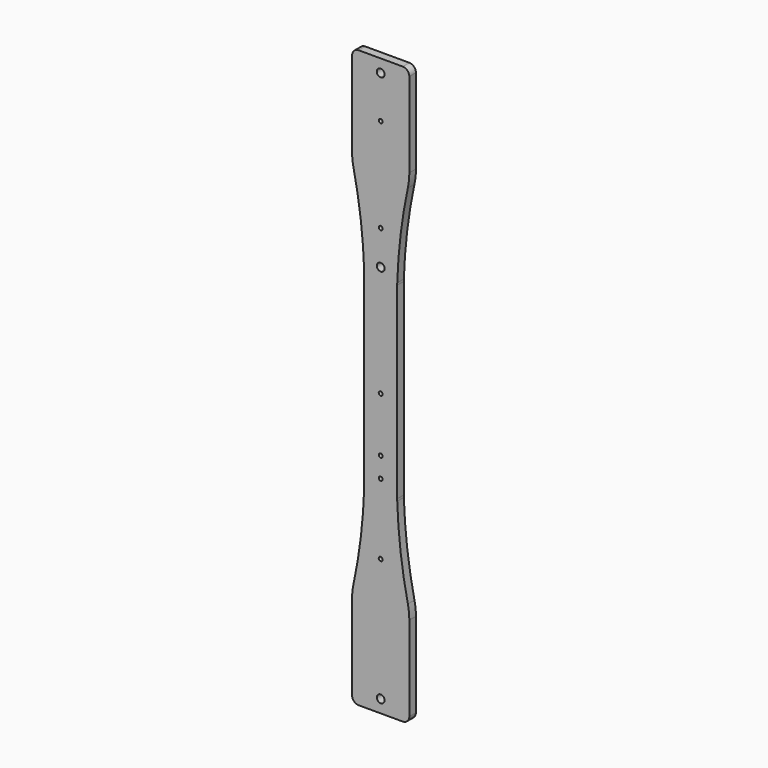
from build123d import *

# Parameters (mm, degrees)
F0_R        = 3
F0_R_2      = 1.5
F1_DEPTH    = 6.35
F2_R        = 5.08
F3_T1_DEPTH = 6.35
F3_T3_DEPTH = 34.0624500619


# Not quite as in the source:
# - a fillet or chamfer that OpenCascade refuses, or shapes differently, is made with other operations: its cross-section is extruded or revolved along the edge and cut away or added
# - a feature names something its author has since deleted; it is built from what else it names


with BuildPart() as f1:
    # F0 (on Front) → F1 (new body)
    with BuildSketch(Plane.XZ):
        with BuildLine():
            Line((-22, -189.9611499309), (-4.6853246795, -189.9611499309))
            Line((-4.6853246795, -189.9611499309), (4.6853246795, -189.9611499309))
            Line((4.6853246795, -189.9611499309), (22, -189.9611499309))
            Line((22, -189.9611499309), (22, -172.8709284505))
            Line((22, -172.8709284505), (22, -114.1058849427))
            ThreePointArc((22, -114.1058849427), (15.5787747464, -77.9579307824), (12.7, -41.3571195934))
            Line((12.7, -41.3571195934), (12.7, 104.7939062119))
            ThreePointArc((12.7, 104.7939062119), (15.5787747464, 141.3947174009), (22, 177.5426715612))
            Line((22, 177.5426715612), (22, 225.4278063774))
            Line((22, 225.4278063774), (22, 236.307715069))
            Line((22, 236.307715069), (22, 253.3979365494))
            Line((22, 253.3979365494), (4.6853246795, 253.3979365494))
            Line((4.6853246795, 253.3979365494), (0, 253.3979365494))
            Line((0, 253.3979365494), (-4.6853246795, 253.3979365494))
            Line((-4.6853246795, 253.3979365494), (-22, 253.3979365494))
            Line((-22, 253.3979365494), (-22, 236.307715069))
            Line((-22, 236.307715069), (-22, 225.4278063774))
            Line((-22, 225.4278063774), (-22, 177.5426715612))
            ThreePointArc((-22, 177.5426715612), (-15.5787747464, 141.3947174009), (-12.7, 104.7939062119))
            Line((-12.7, 104.7939062119), (-12.7, -41.3571195934))
            ThreePointArc((-12.7, -41.3571195934), (-15.5787747464, -77.9579307824), (-22, -114.1058849427))
            Line((-22, -114.1058849427), (-22, -161.9910197589))
            Line((-22, -161.9910197589), (-22, -189.9611499309))
        make_face()
        with Locations((0, -180.0831407309)):
            Circle(F0_R, mode=Mode.SUBTRACT)
        with Locations((0, -85.4520261312)):
            Circle(F0_R_2, mode=Mode.SUBTRACT)
        with Locations((0, -31.0690756887)):
            Circle(F0_R_2, mode=Mode.SUBTRACT)
        with Locations((0, -15.4758756887)):
            Circle(F0_R_2, mode=Mode.SUBTRACT)
        with Locations((0, 26.5547856688)):
            Circle(F0_R_2, mode=Mode.SUBTRACT)
        with BuildLine():
            ThreePointArc((0, 109.0876222849), (-3, 112.0876222849), (0, 115.0876222849))
            ThreePointArc((0, 115.0876222849), (2.1213203436, 114.2089426284), (3, 112.0876222849))
            ThreePointArc((3, 112.0876222849), (2.1213203436, 109.9663019413), (0, 109.0876222849))
        make_face(mode=Mode.SUBTRACT)
        with BuildLine():
            ThreePointArc((0, 137.0615974688), (-1.5, 138.5615974688), (0, 140.0615974688))
            ThreePointArc((0, 140.0615974688), (1.0606601718, 139.6222576406), (1.5, 138.5615974688))
            ThreePointArc((1.5, 138.5615974688), (1.0606601718, 137.5009372971), (0, 137.0615974688))
        make_face(mode=Mode.SUBTRACT)
        with BuildLine():
            ThreePointArc((0, 209.4587856688), (-1.5, 210.9587856688), (0, 212.4587856688))
            ThreePointArc((0, 212.4587856688), (1.0606601718, 212.0194458406), (1.5, 210.9587856688))
            ThreePointArc((1.5, 210.9587856688), (1.0606601718, 209.8981254971), (0, 209.4587856688))
        make_face(mode=Mode.SUBTRACT)
        with BuildLine():
            ThreePointArc((0, 240.5199192026), (-3, 243.5199192026), (0, 246.5199192026))
            ThreePointArc((0, 246.5199192026), (2.1213203436, 245.6412395461), (3, 243.5199192026))
            ThreePointArc((3, 243.5199192026), (2.1213203436, 241.398598859), (0, 240.5199192026))
        make_face(mode=Mode.SUBTRACT)
    extrude(amount=F1_DEPTH)

    # F2
    f2_edges = [f1.edges().sort_by_distance(p)[0] for p in [
        (-22, -3.175, 253.397937),
        (22, -3.175, 253.397937),
        (22, -3.175, -189.96115),
        (-22, -3.175, -189.96115),
    ]]
    fillet(f2_edges, radius=F2_R)

    # F3: fillet of radius 50.8 on 8 edges, made by hand

    # F3_s2 → F3_t1 (join)
    with BuildSketch(Plane.XZ):
        with BuildLine():
            ThreePointArc((-12.7, 104.0086355302), (-12.7065317021, 104.8232386677), (-12.7261251288, 105.6376323271))
            ThreePointArc((-12.7261251288, 105.6376323271), (-12.7128266876, 105.2157765732), (-12.7, 104.7939062119))
            Line((-12.7, 104.7939062119), (-12.7, 104.0086355302))
        make_face()
        with BuildLine():
            ThreePointArc((12.7, 104.0086355302), (12.7065317021, 104.8232386677), (12.7261251288, 105.6376323271))
            ThreePointArc((12.7261251288, 105.6376323271), (12.7128266876, 105.2157765732), (12.7, 104.7939062119))
            Line((12.7, 104.7939062119), (12.7, 104.0086355302))
        make_face()
        with BuildLine():
            ThreePointArc((12.7261251288, -42.2008457086), (12.7065317021, -41.3864520492), (12.7, -40.5718489117))
            Line((12.7, -40.5718489117), (12.7, -41.3571195934))
            ThreePointArc((12.7, -41.3571195934), (12.7128266876, -41.7789899547), (12.7261251288, -42.2008457086))
        make_face()
        with BuildLine():
            ThreePointArc((-12.7261251288, -42.2008457086), (-12.7065317021, -41.3864520492), (-12.7, -40.5718489116))
            Line((-12.7, -40.5718489116), (-12.7, -41.3571195934))
            ThreePointArc((-12.7, -41.3571195934), (-12.7128266876, -41.7789899547), (-12.7261251288, -42.2008457086))
        make_face()
    extrude(amount=F3_T1_DEPTH)

    # F3_s4 → F3_t3 (cut)
    with BuildSketch(Plane.XZ.offset(-13.856225031)):
        with BuildLine():
            ThreePointArc((-22, -119.6483749551), (-21.7184280188, -114.3071737314), (-20.8768334444, -109.025182453))
            ThreePointArc((-20.8768334444, -109.025182453), (-21.429661091, -111.5674692633), (-22, -114.1058849427))
            Line((-22, -114.1058849427), (-22, -119.6483749551))
        make_face()
        with BuildLine():
            ThreePointArc((22, -119.6483749551), (21.7184280188, -114.3071737314), (20.8768334444, -109.025182453))
            ThreePointArc((20.8768334444, -109.025182453), (21.429661091, -111.5674692633), (22, -114.1058849427))
            Line((22, -114.1058849427), (22, -119.6483749551))
        make_face()
        with BuildLine():
            ThreePointArc((20.8768334444, 172.4619690715), (21.7184280188, 177.7439603499), (22, 183.0851615736))
            Line((22, 183.0851615736), (22, 177.5426715612))
            ThreePointArc((22, 177.5426715612), (21.429661091, 175.0042558818), (20.8768334444, 172.4619690715))
        make_face()
        with BuildLine():
            ThreePointArc((-20.8768334444, 172.4619690715), (-21.7184280188, 177.7439603499), (-22, 183.0851615736))
            Line((-22, 183.0851615736), (-22, 177.5426715612))
            ThreePointArc((-22, 177.5426715612), (-21.429661091, 175.0042558818), (-20.8768334444, 172.4619690715))
        make_face()
    extrude(amount=F3_T3_DEPTH, mode=Mode.SUBTRACT)


solid = f1.part
